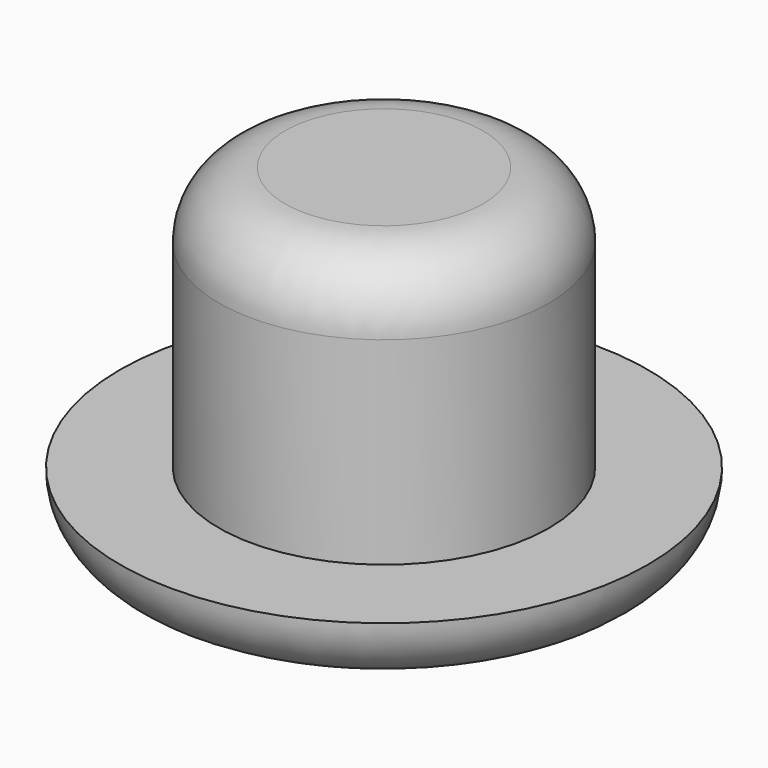
from build123d import *

# Parameters (mm, degrees)
F0_R     = 2.5
F1_DEPTH = 5
F0_R_2   = 4
F2_DEPTH = 1
F3_R     = 0.99999


# Not quite as in the source:
# - a fillet or chamfer is up to 0.001 mm smaller than in the source, because OpenCascade refuses the exact size


with BuildPart() as f1:
    # F0 (on Top) → F1 (new body)
    with BuildSketch(Plane.XY):
        Circle(F0_R)
    extrude(amount=F1_DEPTH)

    # F0 (on Top) → F2 (join)
    with BuildSketch(Plane.XY):
        Circle(F0_R_2)
        Circle(F0_R, mode=Mode.SUBTRACT)
    extrude(amount=F2_DEPTH)

    # F3 (radius 1 in the source; OpenCascade refuses exactly that, so slightly less here)
    f3_edges = [f1.edges().sort_by_distance(p)[0] for p in [
        (-4, 0, 0),
        (-2.5, 0, 5),
    ]]
    fillet(f3_edges, radius=F3_R)


solid = f1.part
